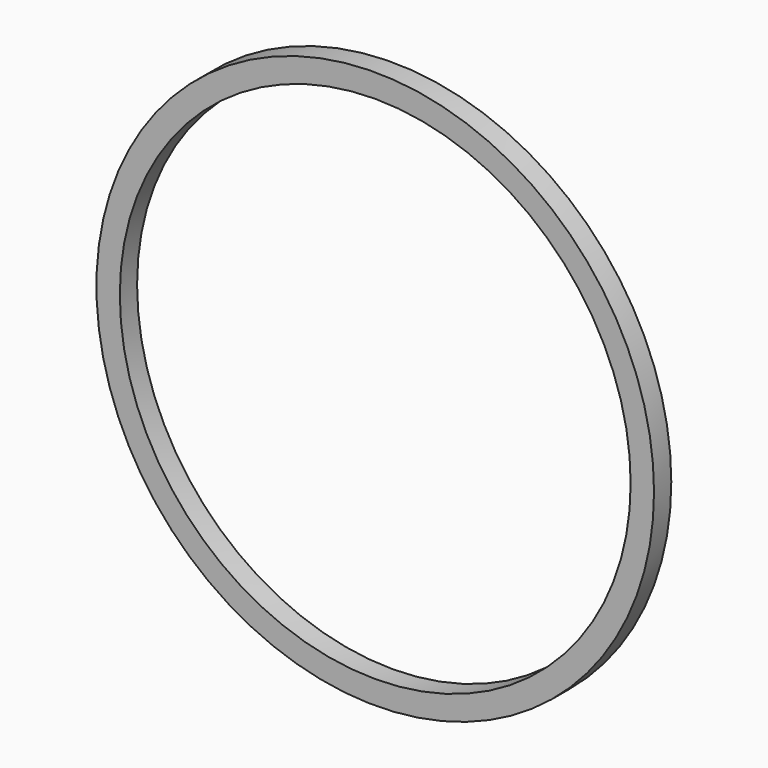
from build123d import *

# Parameters (mm, degrees)
F0_R     = 123.03125
F0_R_2   = 112.7125
F1_DEPTH = 9.525


# Not quite as in the source:
# - a length typed as a fraction of an inch, garbled in the dataset ("3 / 203.2 mm" for 3/8 in), is restored


with BuildPart() as f1:
    # F0 (on Front) → F1 (new body)
    with BuildSketch(Plane.XZ):
        Circle(F0_R)
        Circle(F0_R_2, mode=Mode.SUBTRACT)
    extrude(amount=F1_DEPTH)


solid = f1.part
